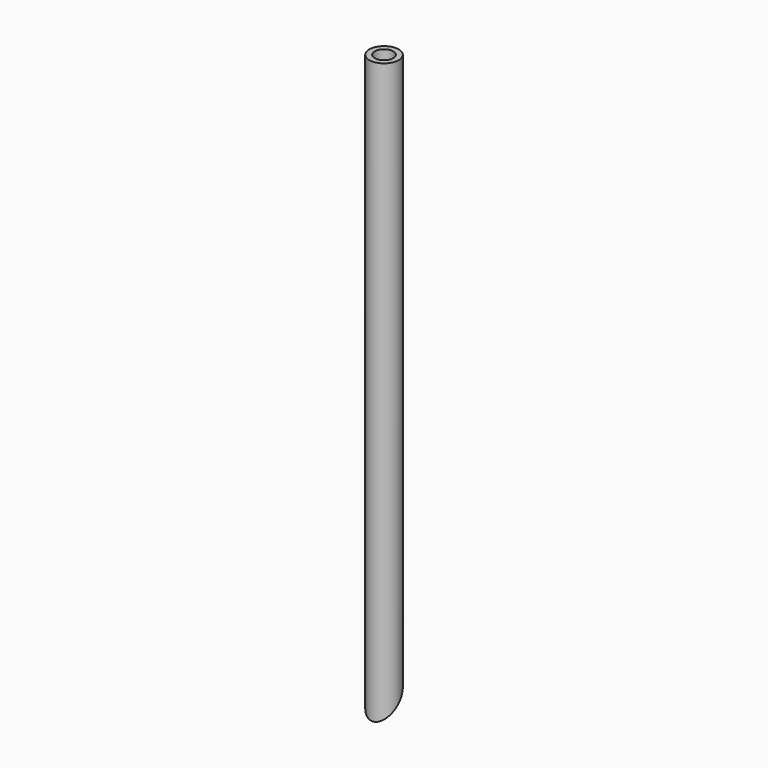
from build123d import *

# Parameters (mm, degrees)
F0_R     = 3
F1_DEPTH = 130
F2_T     = -1.1
F5_R     = 26.2587558367
F6_DEPTH = 25


with BuildPart() as f1:
    # F0 (on Top) → F1 (new body)
    with BuildSketch(Plane.XY):
        Circle(F0_R)
    extrude(amount=F1_DEPTH)

    # F2
    f2_openings = [f1.faces().sort_by_distance(p)[0] for p in [
        (0, 0, 130),
    ]]
    offset(amount=F2_T, openings=f2_openings)

    # F5 (on face) → F6 (cut)
    with BuildSketch(Plane(origin=(0, -7.0710678119, 7.0710678119), x_dir=(1, 0, 0), z_dir=(0, -0.7071067812, 0.7071067812))):
        Circle(F5_R)
    extrude(amount=-F6_DEPTH, mode=Mode.SUBTRACT)


solid = f1.part
